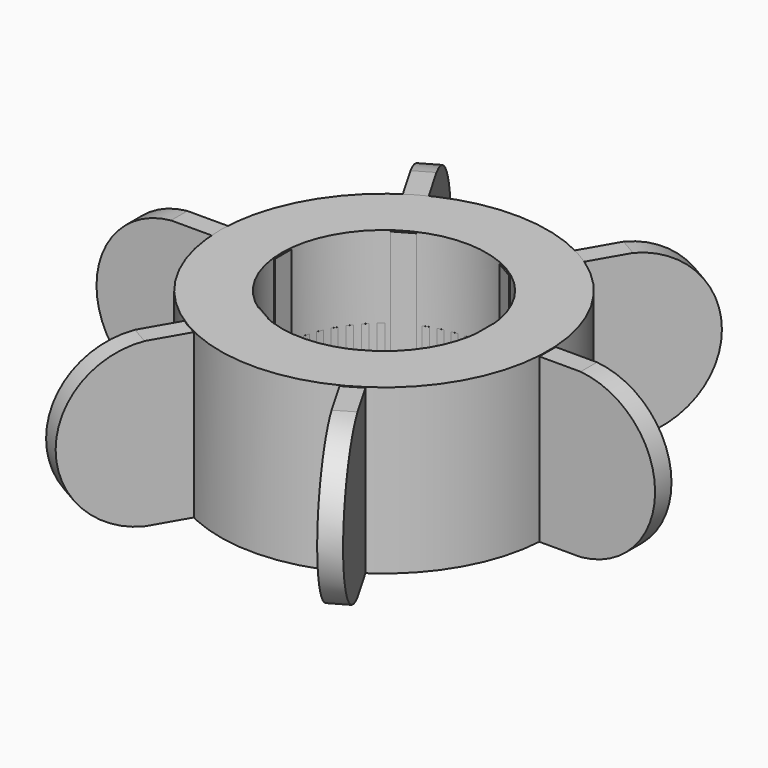
from build123d import *

# Parameters (mm, degrees)
F0_W            = 1
F0_H            = 4
F2_W            = 5.08
F2_H            = 7.9671185657
F3_DEPTH        = 0.5
F3_COPIES_COUNT = 6
F5_W            = 3
F5_H            = 8


# Not quite as in the source:
# - a pattern or mirror of a feature is missing from the dataset's text; its kind, count and spacing are read off the source's solid


with BuildPart() as f1:
    # F0 (on Front) → F1 (revolve)
    with BuildSketch(Plane.XZ):
        with Locations((-5.5, 2)):
            Rectangle(F0_W, F0_H)
    revolve(axis=Axis((0, 0, 19.3039998412), (0, 0, 1)))

    # F2 (on Front) → F3 (join, symmetric)
    with BuildSketch(Plane.XZ):
        with BuildLine():
            Line((-10, 0), (-10, 7.9671185657))
            ThreePointArc((-10, 7.9671185657), (-13.6377080735, 3.9835592829), (-10, 0))
        make_face()
        with Locations((-7.46, 3.9835592829)):
            Rectangle(F2_W, F2_H)
    f3 = extrude(amount=F3_DEPTH, both=True)

    # F3_copies: F3 ×6 about axis
    f3_copies_axis = Axis((0, 0, 0), (0, 0, 1))
    for i in range(1, F3_COPIES_COUNT):
        add(f3.rotate(f3_copies_axis, i * 360 / F3_COPIES_COUNT))


with BuildPart() as f6:
    # F5 (on Front) → F6 (revolve)
    with BuildSketch(Plane.XZ):
        with Locations((-6.5, 4)):
            Rectangle(F5_W, F5_H)
    revolve(axis=Axis((0, 0, 73.8201290369), (0, 0, 1)))


solid = Compound([f1.part, f6.part])
